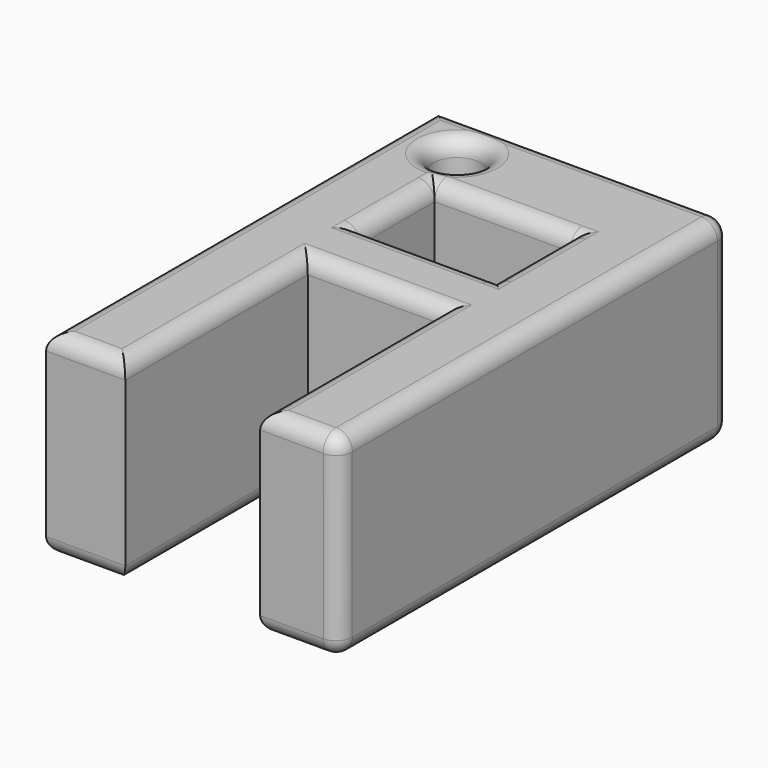
from build123d import *

# Parameters (mm, degrees)
F0_W          = 10.5156756136
F0_H          = 7.2225928307
F1_DEPTH      = 15.24
F2_R          = 1.8806308745
F3_DEPTH      = 25.4
F4_T1_DEPTH   = 24.7648500098
F4_T3_DEPTH   = 35.5602
F4_T5_DEPTH   = 44.4495000197
F4_T7_DEPTH   = 8.0769743963
F4_T9_DEPTH   = 12.5217000197
F4_T11_DEPTH  = 20.9547500098
F4_T13_DEPTH  = 10.5156756136
F4_T15_DEPTH  = 7.2225928307
F4_T17_DEPTH  = 12.7002
F4_S21_W      = 1.2954
F4_S21_H      = 1.2954
F4_T22_DEPTH  = 1.2954
F4_S27_W      = 1.2954
F4_S27_H      = 1.2954
F4_T28_DEPTH  = 1.2954
F4_S33_W      = 1.2954
F4_S33_H      = 1.2954
F4_T34_DEPTH  = 1.2954
F4_S39_W      = 1.2954
F4_S39_H      = 1.2954
F4_T40_DEPTH  = 1.2954
F4_T51_DEPTH  = 24.1295000197
F4_T55_DEPTH  = 13.6904256234
F4_T62_DEPTH  = 24.1295000197
F4_T66_DEPTH  = 13.6904256234
F4_T73_DEPTH  = 13.6904256234
F4_T77_DEPTH  = 10.3973428405
F4_T84_DEPTH  = 13.6904256234
F4_T88_DEPTH  = 10.3973428405
F4_T95_DEPTH  = 10.3973428405
F4_T99_DEPTH  = 13.6904256234
F4_T106_DEPTH = 10.3973428405
F4_T110_DEPTH = 13.6904256234
F4_T117_DEPTH = 24.1295000197
F4_T121_DEPTH = 13.6904256234
F4_T128_DEPTH = 24.1295000197
F4_T132_DEPTH = 13.6904256234
F4_T139_DEPTH = 13.6904256234
F4_T143_DEPTH = 10.3973428405
F4_T150_DEPTH = 13.6904256234
F4_T154_DEPTH = 10.3973428405
F4_T161_DEPTH = 10.3973428405
F4_T165_DEPTH = 13.6904256234
F4_T172_DEPTH = 10.3973428405
F4_T176_DEPTH = 13.6904256234


# Not quite as in the source:
# - a fillet or chamfer that OpenCascade refuses, or shapes differently, is made with other operations: its cross-section is extruded or revolved along the edge and cut away or added


with BuildPart() as f1:
    # F0 (on Top) → F1 (new body)
    with BuildSketch(Plane.XY):
        Polygon((-36.2111851573, 38.1), (-36.2111851573, 0), (-30.0389851573, 0), (-30.0389851573, 17.78), (-19.5233095437, 17.78), (-19.5233095437, 0), (-13.3511851573, 0), (-13.3511851573, 38.1), align=None)
        with Locations((-24.7811473505, 26.5260804445)):
            Rectangle(F0_W, F0_H, mode=Mode.SUBTRACT)
    extrude(amount=F1_DEPTH)

    # F2 (on face) → F3 (cut)
    with BuildSketch(Plane.XY.offset(15.24)):
        with Locations((-31.4282216132, 34.0683087707)):
            Circle(F2_R)
    extrude(amount=-F3_DEPTH, mode=Mode.SUBTRACT)

    # F4: fillet of radius 1.27 on 28 edges, made by hand

    # F4_s2 → F4_t1 (cut)
    with BuildSketch(Plane.YZ.offset(-39.3859351671)):
        with BuildLine():
            ThreePointArc((38.1001, 13.9701), (37.7281256121, 14.8681256121), (36.8301, 15.2401))
            Line((36.8301, 15.2401), (36.8301, 15.2655))
            ThreePointArc((36.8301, 15.2655), (37.46505, 15.2654), (38.1, 15.2654))
            Line((38.1, 15.2654), (38.1254, 15.24))
            ThreePointArc((38.1254, 15.24), (38.1254, 14.60505), (38.1255, 13.9701))
            Line((38.1255, 13.9701), (38.1001, 13.9701))
        make_face()
        with BuildLine():
            ThreePointArc((38.1001, 1.2699), (37.7281256121, 0.3718743879), (36.8301, -0.0001))
            Line((36.8301, -0.0001), (36.8301, -0.0255))
            ThreePointArc((36.8301, -0.0255), (37.46505, -0.0254), (38.1, -0.0254))
            Line((38.1, -0.0254), (38.1254, 0))
            ThreePointArc((38.1254, 0), (38.1254, 0.63495), (38.1255, 1.2699))
            Line((38.1255, 1.2699), (38.1001, 1.2699))
        make_face()
    extrude(amount=F4_T1_DEPTH, mode=Mode.SUBTRACT)

    # F4_s4 → F4_t3 (cut)
    with BuildSketch(Plane.XZ.offset(-36.8301)):
        with BuildLine():
            ThreePointArc((-13.3510851573, 13.9701), (-13.7230595452, 14.8681256121), (-14.6210851573, 15.2401))
            Line((-14.6210851573, 15.2401), (-14.6210851573, 15.2655))
            ThreePointArc((-14.6210851573, 15.2655), (-13.9861351573, 15.2654), (-13.3511851573, 15.2654))
            Line((-13.3511851573, 15.2654), (-13.3257851573, 15.24))
            ThreePointArc((-13.3257851573, 15.24), (-13.3257851573, 14.60505), (-13.3256851573, 13.9701))
            Line((-13.3256851573, 13.9701), (-13.3510851573, 13.9701))
        make_face()
        with BuildLine():
            ThreePointArc((-13.3510851573, 1.2699), (-13.7230595452, 0.3718743879), (-14.6210851573, -0.0001))
            Line((-14.6210851573, -0.0001), (-14.6210851573, -0.0255))
            ThreePointArc((-14.6210851573, -0.0255), (-13.9861351573, -0.0254), (-13.3511851573, -0.0254))
            Line((-13.3511851573, -0.0254), (-13.3257851573, 0))
            ThreePointArc((-13.3257851573, 0), (-13.3257851573, 0.63495), (-13.3256851573, 1.2699))
            Line((-13.3256851573, 1.2699), (-13.3510851573, 1.2699))
        make_face()
    extrude(amount=F4_T3_DEPTH, mode=Mode.SUBTRACT)

    # F4_s6 → F4_t5 (cut)
    with BuildSketch(Plane.XZ.offset(-41.2747500098)):
        with BuildLine():
            ThreePointArc((-36.2112851573, 13.9701), (-35.8393107694, 14.8681256121), (-34.9412851573, 15.2401))
            Line((-34.9412851573, 15.2401), (-34.9412851573, 15.2655))
            ThreePointArc((-34.9412851573, 15.2655), (-35.5762351573, 15.2654), (-36.2111851573, 15.2654))
            Line((-36.2111851573, 15.2654), (-36.2365851573, 15.24))
            ThreePointArc((-36.2365851573, 15.24), (-36.2365851573, 14.60505), (-36.2366851573, 13.9701))
            Line((-36.2366851573, 13.9701), (-36.2112851573, 13.9701))
        make_face()
        with BuildLine():
            ThreePointArc((-36.2112851573, 1.2699), (-35.8393107694, 0.3718743879), (-34.9412851573, -0.0001))
            Line((-34.9412851573, -0.0001), (-34.9412851573, -0.0255))
            ThreePointArc((-34.9412851573, -0.0255), (-35.5762351573, -0.0254), (-36.2111851573, -0.0254))
            Line((-36.2111851573, -0.0254), (-36.2365851573, 0))
            ThreePointArc((-36.2365851573, 0), (-36.2365851573, 0.63495), (-36.2366851573, 1.2699))
            Line((-36.2366851573, 1.2699), (-36.2112851573, 1.2699))
        make_face()
    extrude(amount=F4_T5_DEPTH, mode=Mode.SUBTRACT)

    # F4_s8 → F4_t7 (cut)
    with BuildSketch(Plane.YZ.offset(-22.6980595536)):
        with BuildLine():
            ThreePointArc((1.2699, 15.2401), (0.3718743879, 14.8681256121), (-0.0001, 13.9701))
            Line((-0.0001, 13.9701), (-0.0255, 13.9701))
            ThreePointArc((-0.0255, 13.9701), (-0.0254, 14.60505), (-0.0254, 15.24))
            Line((-0.0254, 15.24), (0, 15.2654))
            ThreePointArc((0, 15.2654), (0.63495, 15.2654), (1.2699, 15.2655))
            Line((1.2699, 15.2655), (1.2699, 15.2401))
        make_face()
        with BuildLine():
            ThreePointArc((1.2699, -0.0001), (0.3718743879, 0.3718743879), (-0.0001, 1.2699))
            Line((-0.0001, 1.2699), (-0.0255, 1.2699))
            ThreePointArc((-0.0255, 1.2699), (-0.0254, 0.63495), (-0.0254, 0))
            Line((-0.0254, 0), (0, -0.0254))
            ThreePointArc((0, -0.0254), (0.63495, -0.0254), (1.2699, -0.0255))
            Line((1.2699, -0.0255), (1.2699, -0.0001))
        make_face()
    extrude(amount=F4_T7_DEPTH, mode=Mode.SUBTRACT)

    # F4_s10 → F4_t9 (cut)
    with BuildSketch(Plane.YZ.offset(-39.3859351671)):
        with BuildLine():
            ThreePointArc((1.2699, 15.2401), (0.3718743879, 14.8681256121), (-0.0001, 13.9701))
            Line((-0.0001, 13.9701), (-0.0255, 13.9701))
            ThreePointArc((-0.0255, 13.9701), (-0.0254, 14.60505), (-0.0254, 15.24))
            Line((-0.0254, 15.24), (0, 15.2654))
            ThreePointArc((0, 15.2654), (0.63495, 15.2654), (1.2699, 15.2655))
            Line((1.2699, 15.2655), (1.2699, 15.2401))
        make_face()
        with BuildLine():
            ThreePointArc((1.2699, -0.0001), (0.3718743879, 0.3718743879), (-0.0001, 1.2699))
            Line((-0.0001, 1.2699), (-0.0255, 1.2699))
            ThreePointArc((-0.0255, 1.2699), (-0.0254, 0.63495), (-0.0254, 0))
            Line((-0.0254, 0), (0, -0.0254))
            ThreePointArc((0, -0.0254), (0.63495, -0.0254), (1.2699, -0.0255))
            Line((1.2699, -0.0255), (1.2699, -0.0001))
        make_face()
    extrude(amount=F4_T9_DEPTH, mode=Mode.SUBTRACT)

    # F4_s12 → F4_t11 (cut)
    with BuildSketch(Plane.XZ.offset(-17.78)):
        with BuildLine():
            ThreePointArc((-18.2534095437, 15.2401), (-19.1514351558, 14.8681256121), (-19.5234095437, 13.9701))
            Line((-19.5234095437, 13.9701), (-19.5488095437, 13.9701))
            ThreePointArc((-19.5488095437, 13.9701), (-19.5487095437, 14.60505), (-19.5487095437, 15.24))
            Line((-19.5487095437, 15.24), (-19.5233095437, 15.2654))
            ThreePointArc((-19.5233095437, 15.2654), (-18.8883595437, 15.2654), (-18.2534095437, 15.2655))
            Line((-18.2534095437, 15.2655), (-18.2534095437, 15.2401))
        make_face()
        with BuildLine():
            ThreePointArc((-31.3088851573, 15.2401), (-30.4108595452, 14.8681256121), (-30.0388851573, 13.9701))
            Line((-30.0388851573, 13.9701), (-30.0134851573, 13.9701))
            ThreePointArc((-30.0134851573, 13.9701), (-30.0135851573, 14.60505), (-30.0135851573, 15.24))
            Line((-30.0135851573, 15.24), (-30.0389851573, 15.2654))
            ThreePointArc((-30.0389851573, 15.2654), (-30.6739351573, 15.2654), (-31.3088851573, 15.2655))
            Line((-31.3088851573, 15.2655), (-31.3088851573, 15.2401))
        make_face()
        with BuildLine():
            ThreePointArc((-18.2534095437, -0.0001), (-19.1514351558, 0.3718743879), (-19.5234095437, 1.2699))
            Line((-19.5234095437, 1.2699), (-19.5488095437, 1.2699))
            ThreePointArc((-19.5488095437, 1.2699), (-19.5487095437, 0.63495), (-19.5487095437, 0))
            Line((-19.5487095437, 0), (-19.5233095437, -0.0254))
            ThreePointArc((-19.5233095437, -0.0254), (-18.8883595437, -0.0254), (-18.2534095437, -0.0255))
            Line((-18.2534095437, -0.0255), (-18.2534095437, -0.0001))
        make_face()
        with BuildLine():
            ThreePointArc((-31.3088851573, -0.0001), (-30.4108595452, 0.3718743879), (-30.0388851573, 1.2699))
            Line((-30.0388851573, 1.2699), (-30.0134851573, 1.2699))
            ThreePointArc((-30.0134851573, 1.2699), (-30.0135851573, 0.63495), (-30.0135851573, 0))
            Line((-30.0135851573, 0), (-30.0389851573, -0.0254))
            ThreePointArc((-30.0389851573, -0.0254), (-30.6739351573, -0.0254), (-31.3088851573, -0.0255))
            Line((-31.3088851573, -0.0255), (-31.3088851573, -0.0001))
        make_face()
    extrude(amount=F4_T11_DEPTH, mode=Mode.SUBTRACT)

    # F4_s14 → F4_t13 (cut)
    with BuildSketch(Plane.YZ.offset(-30.0389851573)):
        with BuildLine():
            ThreePointArc((19.0499, 15.2401), (18.1518743879, 14.8681256121), (17.7799, 13.9701))
            Line((17.7799, 13.9701), (17.7545, 13.9701))
            ThreePointArc((17.7545, 13.9701), (17.7546, 14.60505), (17.7546, 15.24))
            Line((17.7546, 15.24), (17.78, 15.2654))
            ThreePointArc((17.78, 15.2654), (18.41495, 15.2654), (19.0499, 15.2655))
            Line((19.0499, 15.2655), (19.0499, 15.2401))
        make_face()
        with BuildLine():
            ThreePointArc((21.6448840291, 15.2401), (22.5429096412, 14.8681256121), (22.9148840291, 13.9701))
            Line((22.9148840291, 13.9701), (22.9402840291, 13.9701))
            ThreePointArc((22.9402840291, 13.9701), (22.9401840291, 14.60505), (22.9401840291, 15.24))
            Line((22.9401840291, 15.24), (22.9147840291, 15.2654))
            ThreePointArc((22.9147840291, 15.2654), (22.2798340291, 15.2654), (21.6448840291, 15.2655))
            Line((21.6448840291, 15.2655), (21.6448840291, 15.2401))
        make_face()
        with BuildLine():
            ThreePointArc((31.4072768598, 15.2401), (30.5092512477, 14.8681256121), (30.1372768598, 13.9701))
            Line((30.1372768598, 13.9701), (30.1118768598, 13.9701))
            ThreePointArc((30.1118768598, 13.9701), (30.1119768598, 14.60505), (30.1119768598, 15.24))
            Line((30.1119768598, 15.24), (30.1373768598, 15.2654))
            ThreePointArc((30.1373768598, 15.2654), (30.7723268598, 15.2654), (31.4072768598, 15.2655))
            Line((31.4072768598, 15.2655), (31.4072768598, 15.2401))
        make_face()
        with BuildLine():
            ThreePointArc((19.0499, -0.0001), (18.1518743879, 0.3718743879), (17.7799, 1.2699))
            Line((17.7799, 1.2699), (17.7545, 1.2699))
            ThreePointArc((17.7545, 1.2699), (17.7546, 0.63495), (17.7546, 0))
            Line((17.7546, 0), (17.78, -0.0254))
            ThreePointArc((17.78, -0.0254), (18.41495, -0.0254), (19.0499, -0.0255))
            Line((19.0499, -0.0255), (19.0499, -0.0001))
        make_face()
        with BuildLine():
            ThreePointArc((21.6448840291, -0.0001), (22.5429096412, 0.3718743879), (22.9148840291, 1.2699))
            Line((22.9148840291, 1.2699), (22.9402840291, 1.2699))
            ThreePointArc((22.9402840291, 1.2699), (22.9401840291, 0.63495), (22.9401840291, 0))
            Line((22.9401840291, 0), (22.9147840291, -0.0254))
            ThreePointArc((22.9147840291, -0.0254), (22.2798340291, -0.0254), (21.6448840291, -0.0255))
            Line((21.6448840291, -0.0255), (21.6448840291, -0.0001))
        make_face()
        with BuildLine():
            ThreePointArc((31.4072768598, -0.0001), (30.5092512477, 0.3718743879), (30.1372768598, 1.2699))
            Line((30.1372768598, 1.2699), (30.1118768598, 1.2699))
            ThreePointArc((30.1118768598, 1.2699), (30.1119768598, 0.63495), (30.1119768598, 0))
            Line((30.1119768598, 0), (30.1373768598, -0.0254))
            ThreePointArc((30.1373768598, -0.0254), (30.7723268598, -0.0254), (31.4072768598, -0.0255))
            Line((31.4072768598, -0.0255), (31.4072768598, -0.0001))
        make_face()
    extrude(amount=F4_T13_DEPTH, mode=Mode.SUBTRACT)

    # F4_s16 → F4_t15 (cut)
    with BuildSketch(Plane.XZ.offset(-30.1373768598)):
        with BuildLine():
            ThreePointArc((-18.2534095437, 15.2401), (-19.1514351558, 14.8681256121), (-19.5234095437, 13.9701))
            Line((-19.5234095437, 13.9701), (-19.5488095437, 13.9701))
            ThreePointArc((-19.5488095437, 13.9701), (-19.5487095437, 14.60505), (-19.5487095437, 15.24))
            Line((-19.5487095437, 15.24), (-19.5233095437, 15.2654))
            ThreePointArc((-19.5233095437, 15.2654), (-18.8883595437, 15.2654), (-18.2534095437, 15.2655))
            Line((-18.2534095437, 15.2655), (-18.2534095437, 15.2401))
        make_face()
        with BuildLine():
            ThreePointArc((-31.3088851573, 15.2401), (-30.4108595452, 14.8681256121), (-30.0388851573, 13.9701))
            Line((-30.0388851573, 13.9701), (-30.0134851573, 13.9701))
            ThreePointArc((-30.0134851573, 13.9701), (-30.0135851573, 14.60505), (-30.0135851573, 15.24))
            Line((-30.0135851573, 15.24), (-30.0389851573, 15.2654))
            ThreePointArc((-30.0389851573, 15.2654), (-30.6739351573, 15.2654), (-31.3088851573, 15.2655))
            Line((-31.3088851573, 15.2655), (-31.3088851573, 15.2401))
        make_face()
        with BuildLine():
            ThreePointArc((-18.2534095437, -0.0001), (-19.1514351558, 0.3718743879), (-19.5234095437, 1.2699))
            Line((-19.5234095437, 1.2699), (-19.5488095437, 1.2699))
            ThreePointArc((-19.5488095437, 1.2699), (-19.5487095437, 0.63495), (-19.5487095437, 0))
            Line((-19.5487095437, 0), (-19.5233095437, -0.0254))
            ThreePointArc((-19.5233095437, -0.0254), (-18.8883595437, -0.0254), (-18.2534095437, -0.0255))
            Line((-18.2534095437, -0.0255), (-18.2534095437, -0.0001))
        make_face()
        with BuildLine():
            ThreePointArc((-31.3088851573, -0.0001), (-30.4108595452, 0.3718743879), (-30.0388851573, 1.2699))
            Line((-30.0388851573, 1.2699), (-30.0134851573, 1.2699))
            ThreePointArc((-30.0134851573, 1.2699), (-30.0135851573, 0.63495), (-30.0135851573, 0))
            Line((-30.0135851573, 0), (-30.0389851573, -0.0254))
            ThreePointArc((-30.0389851573, -0.0254), (-30.6739351573, -0.0254), (-31.3088851573, -0.0255))
            Line((-31.3088851573, -0.0255), (-31.3088851573, -0.0001))
        make_face()
    extrude(amount=F4_T15_DEPTH, mode=Mode.SUBTRACT)

    # F4_s18 → F4_t17 (cut)
    with BuildSketch(Plane.XY.offset(1.2699)):
        with BuildLine():
            ThreePointArc((-13.3510851573, 1.2699), (-13.7230595452, 0.3718743879), (-14.6210851573, -0.0001))
            Line((-14.6210851573, -0.0001), (-14.6210851573, -0.0255))
            ThreePointArc((-14.6210851573, -0.0255), (-13.9861351573, -0.0254), (-13.3511851573, -0.0254))
            Line((-13.3511851573, -0.0254), (-13.3257851573, 0))
            ThreePointArc((-13.3257851573, 0), (-13.3257851573, 0.63495), (-13.3256851573, 1.2699))
            Line((-13.3256851573, 1.2699), (-13.3510851573, 1.2699))
        make_face()
        with BuildLine():
            ThreePointArc((-14.6210851573, 38.1001), (-13.7230595452, 37.7281256121), (-13.3510851573, 36.8301))
            Line((-13.3510851573, 36.8301), (-13.3256851573, 36.8301))
            ThreePointArc((-13.3256851573, 36.8301), (-13.3257851573, 37.46505), (-13.3257851573, 38.1))
            Line((-13.3257851573, 38.1), (-13.3511851573, 38.1254))
            ThreePointArc((-13.3511851573, 38.1254), (-13.9861351573, 38.1254), (-14.6210851573, 38.1255))
            Line((-14.6210851573, 38.1255), (-14.6210851573, 38.1001))
        make_face()
    extrude(amount=F4_T17_DEPTH, mode=Mode.SUBTRACT)


with BuildPart() as f4_tool20:
    # F4_s21 → F4_t22 (new body)
    with BuildSketch(Plane.XZ.offset(-36.8301)):
        with Locations((-13.9733851573, 14.6178)):
            Rectangle(F4_S21_W, F4_S21_H)
    extrude(amount=-F4_T22_DEPTH)

    # F4_s23 → F4_t24 (revolve, cut)
    with BuildSketch(Plane(origin=(-14.6210851573, 36.8301, 13.9701), x_dir=(-0.7071067812, 0, -0.7071067812), z_dir=(0.7071067812, 0, -0.7071067812))):
        with BuildLine():
            ThreePointArc((0, -1.27), (1.27, 0), (0, 1.27))
            Line((0, 1.27), (0, -1.27))
        make_face()
    revolve(axis=Axis((-14.6210851573, 36.8301, 13.9701), (0, 1, 0)), mode=Mode.SUBTRACT)


with BuildPart() as f1_1:
    add(f1.part)

    # F4_t19: cut F4_tool20
    add(f4_tool20.part, mode=Mode.SUBTRACT)


with BuildPart() as f4_tool26:
    # F4_s27 → F4_t28 (new body)
    with BuildSketch(Plane.YZ.offset(-14.6210851573)):
        with Locations((0.6222, 14.6178)):
            Rectangle(F4_S27_W, F4_S27_H)
    extrude(amount=F4_T28_DEPTH)

    # F4_s29 → F4_t30 (revolve, cut)
    with BuildSketch(Plane(origin=(-14.6210851573, 1.2699, 13.9701), x_dir=(0, 0.7071067812, -0.7071067812), z_dir=(0, -0.7071067812, -0.7071067812))):
        with BuildLine():
            ThreePointArc((0, -1.27), (1.27, 0), (0, 1.27))
            Line((0, 1.27), (0, -1.27))
        make_face()
    revolve(axis=Axis((-14.6210851573, 1.2699, 13.9701), (1, 0, 0)), mode=Mode.SUBTRACT)


with BuildPart() as f1_2:
    add(f1_1.part)

    # F4_t25: cut F4_tool26
    add(f4_tool26.part, mode=Mode.SUBTRACT)


with BuildPart() as f4_tool32:
    # F4_s33 → F4_t34 (new body)
    with BuildSketch(Plane.XZ.offset(-36.8301)):
        with Locations((-13.9733851573, 0.6222)):
            Rectangle(F4_S33_W, F4_S33_H)
    extrude(amount=-F4_T34_DEPTH)

    # F4_s35 → F4_t36 (revolve, cut)
    with BuildSketch(Plane(origin=(-14.6210851573, 36.8301, 1.2699), x_dir=(-0.7071067812, 0, 0.7071067812), z_dir=(-0.7071067812, 0, -0.7071067812))):
        with BuildLine():
            ThreePointArc((0, -1.27), (1.27, 0), (0, 1.27))
            Line((0, 1.27), (0, -1.27))
        make_face()
    revolve(axis=Axis((-14.6210851573, 36.8301, 1.2699), (0, 1, 0)), mode=Mode.SUBTRACT)


with BuildPart() as f1_3:
    add(f1_2.part)

    # F4_t31: cut F4_tool32
    add(f4_tool32.part, mode=Mode.SUBTRACT)


with BuildPart() as f4_tool38:
    # F4_s39 → F4_t40 (new body)
    with BuildSketch(Plane.YZ.offset(-14.6210851573)):
        with Locations((0.6222, 0.6222)):
            Rectangle(F4_S39_W, F4_S39_H)
    extrude(amount=F4_T40_DEPTH)

    # F4_s41 → F4_t42 (revolve, cut)
    with BuildSketch(Plane(origin=(-14.6210851573, 1.2699, 1.2699), x_dir=(0, 0.7071067812, 0.7071067812), z_dir=(0, 0.7071067812, -0.7071067812))):
        with BuildLine():
            ThreePointArc((0, -1.27), (1.27, 0), (0, 1.27))
            Line((0, 1.27), (0, -1.27))
        make_face()
    revolve(axis=Axis((-14.6210851573, 1.2699, 1.2699), (1, 0, 0)), mode=Mode.SUBTRACT)


with BuildPart() as f1_4:
    add(f1_3.part)

    # F4_t37: cut F4_tool38
    add(f4_tool38.part, mode=Mode.SUBTRACT)

    # F4_s43 → F4_t44 (revolve, cut)
    with BuildSketch(Plane.XZ.offset(-34.0683087707)):
        with BuildLine():
            ThreePointArc((-28.2776907386, 15.2401), (-29.1757163507, 14.8681256121), (-29.5476907386, 13.9701))
            Line((-29.5476907386, 13.9701), (-29.5730907386, 13.9701))
            ThreePointArc((-29.5730907386, 13.9701), (-29.5729907386, 14.60505), (-29.5729907386, 15.24))
            Line((-29.5729907386, 15.24), (-29.5475907386, 15.2654))
            ThreePointArc((-29.5475907386, 15.2654), (-28.9126407386, 15.2654), (-28.2776907386, 15.2655))
            Line((-28.2776907386, 15.2655), (-28.2776907386, 15.2401))
        make_face()
    revolve(axis=Axis((-31.4282216132, 34.0683087707, 15.24), (0, 0, 1)), mode=Mode.SUBTRACT)

    # F4_s45 → F4_t46 (revolve, cut)
    with BuildSketch(Plane.XZ.offset(-34.0683087707)):
        with BuildLine():
            ThreePointArc((-28.2776907386, -0.0001), (-29.1757163507, 0.3718743879), (-29.5476907386, 1.2699))
            Line((-29.5476907386, 1.2699), (-29.5730907386, 1.2699))
            ThreePointArc((-29.5730907386, 1.2699), (-29.5729907386, 0.63495), (-29.5729907386, 0))
            Line((-29.5729907386, 0), (-29.5475907386, -0.0254))
            ThreePointArc((-29.5475907386, -0.0254), (-28.9126407386, -0.0254), (-28.2776907386, -0.0255))
            Line((-28.2776907386, -0.0255), (-28.2776907386, -0.0001))
        make_face()
    revolve(axis=Axis((-31.4282216132, 34.0683087707, 0), (0, 0, 1)), mode=Mode.SUBTRACT)


with BuildPart() as f4_tool49:
    # F4_s50 → F4_t51 (new body)
    with BuildSketch(Plane.XZ.offset(-20.9547500098)):
        with BuildLine():
            ThreePointArc((-18.2534095437, 15.2401), (-19.1514351558, 14.8681256121), (-19.5234095437, 13.9701))
            Line((-19.5234095437, 13.9701), (-19.5488095437, 13.9701))
            ThreePointArc((-19.5488095437, 13.9701), (-19.5487095437, 14.60505), (-19.5487095437, 15.24))
            Line((-19.5487095437, 15.24), (-19.5233095437, 15.2654))
            ThreePointArc((-19.5233095437, 15.2654), (-18.8883595437, 15.2654), (-18.2534095437, 15.2655))
            Line((-18.2534095437, 15.2655), (-18.2534095437, 15.2401))
        make_face()
    extrude(amount=F4_T51_DEPTH)

    split(bisect_by=Plane.XZ.offset(-17.78), keep=Keep.BOTTOM)


with BuildPart() as f4_tool53:
    # F4_s54 → F4_t55 (new body)
    with BuildSketch(Plane.YZ.offset(-30.0389851573)):
        with BuildLine():
            ThreePointArc((19.0499, 15.2401), (18.1518743879, 14.8681256121), (17.7799, 13.9701))
            Line((17.7799, 13.9701), (17.7545, 13.9701))
            ThreePointArc((17.7545, 13.9701), (17.7546, 14.60505), (17.7546, 15.24))
            Line((17.7546, 15.24), (17.78, 15.2654))
            ThreePointArc((17.78, 15.2654), (18.41495, 15.2654), (19.0499, 15.2655))
            Line((19.0499, 15.2655), (19.0499, 15.2401))
        make_face()
    extrude(amount=F4_T55_DEPTH)

    split(bisect_by=Plane.YZ.offset(-19.5233095437), keep=Keep.TOP)


with BuildPart() as f4_tool49_1:
    add(f4_tool49.part)

    # F4_t57: intersect F4_tool53
    add(f4_tool53.part, mode=Mode.INTERSECT)


with BuildPart() as f1_5:
    add(f1_4.part)

    # F4_t47: cut F4_tool49
    add(f4_tool49_1.part, mode=Mode.SUBTRACT)


with BuildPart() as f4_tool60:
    # F4_s61 → F4_t62 (new body)
    with BuildSketch(Plane.XZ.offset(3.1747500098)):
        with BuildLine():
            ThreePointArc((-31.3088851573, 15.2401), (-30.4108595452, 14.8681256121), (-30.0388851573, 13.9701))
            Line((-30.0388851573, 13.9701), (-30.0134851573, 13.9701))
            ThreePointArc((-30.0134851573, 13.9701), (-30.0135851573, 14.60505), (-30.0135851573, 15.24))
            Line((-30.0135851573, 15.24), (-30.0389851573, 15.2654))
            ThreePointArc((-30.0389851573, 15.2654), (-30.6739351573, 15.2654), (-31.3088851573, 15.2655))
            Line((-31.3088851573, 15.2655), (-31.3088851573, 15.2401))
        make_face()
    extrude(amount=-F4_T62_DEPTH)

    split(bisect_by=Plane.XZ.offset(-17.78), keep=Keep.BOTTOM)


with BuildPart() as f4_tool64:
    # F4_s65 → F4_t66 (new body)
    with BuildSketch(Plane.YZ.offset(-33.2137351671)):
        with BuildLine():
            ThreePointArc((19.0499, 15.2401), (18.1518743879, 14.8681256121), (17.7799, 13.9701))
            Line((17.7799, 13.9701), (17.7545, 13.9701))
            ThreePointArc((17.7545, 13.9701), (17.7546, 14.60505), (17.7546, 15.24))
            Line((17.7546, 15.24), (17.78, 15.2654))
            ThreePointArc((17.78, 15.2654), (18.41495, 15.2654), (19.0499, 15.2655))
            Line((19.0499, 15.2655), (19.0499, 15.2401))
        make_face()
    extrude(amount=F4_T66_DEPTH)

    split(bisect_by=Plane.YZ.offset(-30.0389851573), keep=Keep.BOTTOM)


with BuildPart() as f4_tool60_1:
    add(f4_tool60.part)

    # F4_t68: intersect F4_tool64
    add(f4_tool64.part, mode=Mode.INTERSECT)


with BuildPart() as f1_6:
    add(f1_5.part)

    # F4_t58: cut F4_tool60
    add(f4_tool60_1.part, mode=Mode.SUBTRACT)


with BuildPart() as f4_tool71:
    # F4_s72 → F4_t73 (new body)
    with BuildSketch(Plane.YZ.offset(-16.3485595339)):
        with BuildLine():
            ThreePointArc((21.6448840291, 15.2401), (22.5429096412, 14.8681256121), (22.9148840291, 13.9701))
            Line((22.9148840291, 13.9701), (22.9402840291, 13.9701))
            ThreePointArc((22.9402840291, 13.9701), (22.9401840291, 14.60505), (22.9401840291, 15.24))
            Line((22.9401840291, 15.24), (22.9147840291, 15.2654))
            ThreePointArc((22.9147840291, 15.2654), (22.2798340291, 15.2654), (21.6448840291, 15.2655))
            Line((21.6448840291, 15.2655), (21.6448840291, 15.2401))
        make_face()
    extrude(amount=-F4_T73_DEPTH)

    split(bisect_by=Plane.YZ.offset(-19.5233095437), keep=Keep.TOP)


with BuildPart() as f4_tool75:
    # F4_s76 → F4_t77 (new body)
    with BuildSketch(Plane.XZ.offset(-30.1373768598)):
        with BuildLine():
            ThreePointArc((-18.2534095437, 15.2401), (-19.1514351558, 14.8681256121), (-19.5234095437, 13.9701))
            Line((-19.5234095437, 13.9701), (-19.5488095437, 13.9701))
            ThreePointArc((-19.5488095437, 13.9701), (-19.5487095437, 14.60505), (-19.5487095437, 15.24))
            Line((-19.5487095437, 15.24), (-19.5233095437, 15.2654))
            ThreePointArc((-19.5233095437, 15.2654), (-18.8883595437, 15.2654), (-18.2534095437, 15.2655))
            Line((-18.2534095437, 15.2655), (-18.2534095437, 15.2401))
        make_face()
    extrude(amount=F4_T77_DEPTH)

    split(bisect_by=Plane.XZ.offset(-22.9147840291), keep=Keep.TOP)


with BuildPart() as f4_tool71_1:
    add(f4_tool71.part)

    # F4_t79: intersect F4_tool75
    add(f4_tool75.part, mode=Mode.INTERSECT)


with BuildPart() as f1_7:
    add(f1_6.part)

    # F4_t69: cut F4_tool71
    add(f4_tool71_1.part, mode=Mode.SUBTRACT)


with BuildPart() as f4_tool82:
    # F4_s83 → F4_t84 (new body)
    with BuildSketch(Plane.YZ.offset(-19.5233095437)):
        with BuildLine():
            ThreePointArc((21.6448840291, 15.2401), (22.5429096412, 14.8681256121), (22.9148840291, 13.9701))
            Line((22.9148840291, 13.9701), (22.9402840291, 13.9701))
            ThreePointArc((22.9402840291, 13.9701), (22.9401840291, 14.60505), (22.9401840291, 15.24))
            Line((22.9401840291, 15.24), (22.9147840291, 15.2654))
            ThreePointArc((22.9147840291, 15.2654), (22.2798340291, 15.2654), (21.6448840291, 15.2655))
            Line((21.6448840291, 15.2655), (21.6448840291, 15.2401))
        make_face()
    extrude(amount=-F4_T84_DEPTH)

    split(bisect_by=Plane.YZ.offset(-30.0389851573), keep=Keep.BOTTOM)


with BuildPart() as f4_tool86:
    # F4_s87 → F4_t88 (new body)
    with BuildSketch(Plane.XZ.offset(-19.7400340193)):
        with BuildLine():
            ThreePointArc((-31.3088851573, 15.2401), (-30.4108595452, 14.8681256121), (-30.0388851573, 13.9701))
            Line((-30.0388851573, 13.9701), (-30.0134851573, 13.9701))
            ThreePointArc((-30.0134851573, 13.9701), (-30.0135851573, 14.60505), (-30.0135851573, 15.24))
            Line((-30.0135851573, 15.24), (-30.0389851573, 15.2654))
            ThreePointArc((-30.0389851573, 15.2654), (-30.6739351573, 15.2654), (-31.3088851573, 15.2655))
            Line((-31.3088851573, 15.2655), (-31.3088851573, 15.2401))
        make_face()
    extrude(amount=-F4_T88_DEPTH)

    split(bisect_by=Plane.XZ.offset(-22.9147840291), keep=Keep.TOP)


with BuildPart() as f4_tool82_1:
    add(f4_tool82.part)

    # F4_t90: intersect F4_tool86
    add(f4_tool86.part, mode=Mode.INTERSECT)


with BuildPart() as f1_8:
    add(f1_7.part)

    # F4_t80: cut F4_tool82
    add(f4_tool82_1.part, mode=Mode.SUBTRACT)


with BuildPart() as f4_tool93:
    # F4_s94 → F4_t95 (new body)
    with BuildSketch(Plane.XZ.offset(-33.3121268696)):
        with BuildLine():
            ThreePointArc((-18.2534095437, 15.2401), (-19.1514351558, 14.8681256121), (-19.5234095437, 13.9701))
            Line((-19.5234095437, 13.9701), (-19.5488095437, 13.9701))
            ThreePointArc((-19.5488095437, 13.9701), (-19.5487095437, 14.60505), (-19.5487095437, 15.24))
            Line((-19.5487095437, 15.24), (-19.5233095437, 15.2654))
            ThreePointArc((-19.5233095437, 15.2654), (-18.8883595437, 15.2654), (-18.2534095437, 15.2655))
            Line((-18.2534095437, 15.2655), (-18.2534095437, 15.2401))
        make_face()
    extrude(amount=F4_T95_DEPTH)

    split(bisect_by=Plane.XZ.offset(-30.1373768598), keep=Keep.BOTTOM)


with BuildPart() as f4_tool97:
    # F4_s98 → F4_t99 (new body)
    with BuildSketch(Plane.YZ.offset(-30.0389851573)):
        with BuildLine():
            ThreePointArc((31.4072768598, 15.2401), (30.5092512477, 14.8681256121), (30.1372768598, 13.9701))
            Line((30.1372768598, 13.9701), (30.1118768598, 13.9701))
            ThreePointArc((30.1118768598, 13.9701), (30.1119768598, 14.60505), (30.1119768598, 15.24))
            Line((30.1119768598, 15.24), (30.1373768598, 15.2654))
            ThreePointArc((30.1373768598, 15.2654), (30.7723268598, 15.2654), (31.4072768598, 15.2655))
            Line((31.4072768598, 15.2655), (31.4072768598, 15.2401))
        make_face()
    extrude(amount=F4_T99_DEPTH)

    split(bisect_by=Plane.YZ.offset(-19.5233095437), keep=Keep.TOP)


with BuildPart() as f4_tool93_1:
    add(f4_tool93.part)

    # F4_t101: intersect F4_tool97
    add(f4_tool97.part, mode=Mode.INTERSECT)


with BuildPart() as f1_9:
    add(f1_8.part)

    # F4_t91: cut F4_tool93
    add(f4_tool93_1.part, mode=Mode.SUBTRACT)


with BuildPart() as f4_tool104:
    # F4_s105 → F4_t106 (new body)
    with BuildSketch(Plane.XZ.offset(-22.9147840291)):
        with BuildLine():
            ThreePointArc((-31.3088851573, 15.2401), (-30.4108595452, 14.8681256121), (-30.0388851573, 13.9701))
            Line((-30.0388851573, 13.9701), (-30.0134851573, 13.9701))
            ThreePointArc((-30.0134851573, 13.9701), (-30.0135851573, 14.60505), (-30.0135851573, 15.24))
            Line((-30.0135851573, 15.24), (-30.0389851573, 15.2654))
            ThreePointArc((-30.0389851573, 15.2654), (-30.6739351573, 15.2654), (-31.3088851573, 15.2655))
            Line((-31.3088851573, 15.2655), (-31.3088851573, 15.2401))
        make_face()
    extrude(amount=-F4_T106_DEPTH)

    split(bisect_by=Plane.XZ.offset(-30.1373768598), keep=Keep.BOTTOM)


with BuildPart() as f4_tool108:
    # F4_s109 → F4_t110 (new body)
    with BuildSketch(Plane.YZ.offset(-33.2137351671)):
        with BuildLine():
            ThreePointArc((31.4072768598, 15.2401), (30.5092512477, 14.8681256121), (30.1372768598, 13.9701))
            Line((30.1372768598, 13.9701), (30.1118768598, 13.9701))
            ThreePointArc((30.1118768598, 13.9701), (30.1119768598, 14.60505), (30.1119768598, 15.24))
            Line((30.1119768598, 15.24), (30.1373768598, 15.2654))
            ThreePointArc((30.1373768598, 15.2654), (30.7723268598, 15.2654), (31.4072768598, 15.2655))
            Line((31.4072768598, 15.2655), (31.4072768598, 15.2401))
        make_face()
    extrude(amount=F4_T110_DEPTH)

    split(bisect_by=Plane.YZ.offset(-30.0389851573), keep=Keep.BOTTOM)


with BuildPart() as f4_tool104_1:
    add(f4_tool104.part)

    # F4_t112: intersect F4_tool108
    add(f4_tool108.part, mode=Mode.INTERSECT)


with BuildPart() as f1_10:
    add(f1_9.part)

    # F4_t102: cut F4_tool104
    add(f4_tool104_1.part, mode=Mode.SUBTRACT)


with BuildPart() as f4_tool115:
    # F4_s116 → F4_t117 (new body)
    with BuildSketch(Plane.XZ.offset(-20.9547500098)):
        with BuildLine():
            ThreePointArc((-18.2534095437, -0.0001), (-19.1514351558, 0.3718743879), (-19.5234095437, 1.2699))
            Line((-19.5234095437, 1.2699), (-19.5488095437, 1.2699))
            ThreePointArc((-19.5488095437, 1.2699), (-19.5487095437, 0.63495), (-19.5487095437, 0))
            Line((-19.5487095437, 0), (-19.5233095437, -0.0254))
            ThreePointArc((-19.5233095437, -0.0254), (-18.8883595437, -0.0254), (-18.2534095437, -0.0255))
            Line((-18.2534095437, -0.0255), (-18.2534095437, -0.0001))
        make_face()
    extrude(amount=F4_T117_DEPTH)

    split(bisect_by=Plane.XZ.offset(-17.78), keep=Keep.BOTTOM)


with BuildPart() as f4_tool119:
    # F4_s120 → F4_t121 (new body)
    with BuildSketch(Plane.YZ.offset(-30.0389851573)):
        with BuildLine():
            ThreePointArc((19.0499, -0.0001), (18.1518743879, 0.3718743879), (17.7799, 1.2699))
            Line((17.7799, 1.2699), (17.7545, 1.2699))
            ThreePointArc((17.7545, 1.2699), (17.7546, 0.63495), (17.7546, 0))
            Line((17.7546, 0), (17.78, -0.0254))
            ThreePointArc((17.78, -0.0254), (18.41495, -0.0254), (19.0499, -0.0255))
            Line((19.0499, -0.0255), (19.0499, -0.0001))
        make_face()
    extrude(amount=F4_T121_DEPTH)

    split(bisect_by=Plane.YZ.offset(-19.5233095437), keep=Keep.TOP)


with BuildPart() as f4_tool115_1:
    add(f4_tool115.part)

    # F4_t123: intersect F4_tool119
    add(f4_tool119.part, mode=Mode.INTERSECT)


with BuildPart() as f1_11:
    add(f1_10.part)

    # F4_t113: cut F4_tool115
    add(f4_tool115_1.part, mode=Mode.SUBTRACT)


with BuildPart() as f4_tool126:
    # F4_s127 → F4_t128 (new body)
    with BuildSketch(Plane.XZ.offset(3.1747500098)):
        with BuildLine():
            ThreePointArc((-31.3088851573, -0.0001), (-30.4108595452, 0.3718743879), (-30.0388851573, 1.2699))
            Line((-30.0388851573, 1.2699), (-30.0134851573, 1.2699))
            ThreePointArc((-30.0134851573, 1.2699), (-30.0135851573, 0.63495), (-30.0135851573, 0))
            Line((-30.0135851573, 0), (-30.0389851573, -0.0254))
            ThreePointArc((-30.0389851573, -0.0254), (-30.6739351573, -0.0254), (-31.3088851573, -0.0255))
            Line((-31.3088851573, -0.0255), (-31.3088851573, -0.0001))
        make_face()
    extrude(amount=-F4_T128_DEPTH)

    split(bisect_by=Plane.XZ.offset(-17.78), keep=Keep.BOTTOM)


with BuildPart() as f4_tool130:
    # F4_s131 → F4_t132 (new body)
    with BuildSketch(Plane.YZ.offset(-33.2137351671)):
        with BuildLine():
            ThreePointArc((19.0499, -0.0001), (18.1518743879, 0.3718743879), (17.7799, 1.2699))
            Line((17.7799, 1.2699), (17.7545, 1.2699))
            ThreePointArc((17.7545, 1.2699), (17.7546, 0.63495), (17.7546, 0))
            Line((17.7546, 0), (17.78, -0.0254))
            ThreePointArc((17.78, -0.0254), (18.41495, -0.0254), (19.0499, -0.0255))
            Line((19.0499, -0.0255), (19.0499, -0.0001))
        make_face()
    extrude(amount=F4_T132_DEPTH)

    split(bisect_by=Plane.YZ.offset(-30.0389851573), keep=Keep.BOTTOM)


with BuildPart() as f4_tool126_1:
    add(f4_tool126.part)

    # F4_t134: intersect F4_tool130
    add(f4_tool130.part, mode=Mode.INTERSECT)


with BuildPart() as f1_12:
    add(f1_11.part)

    # F4_t124: cut F4_tool126
    add(f4_tool126_1.part, mode=Mode.SUBTRACT)


with BuildPart() as f4_tool137:
    # F4_s138 → F4_t139 (new body)
    with BuildSketch(Plane.YZ.offset(-16.3485595339)):
        with BuildLine():
            ThreePointArc((21.6448840291, -0.0001), (22.5429096412, 0.3718743879), (22.9148840291, 1.2699))
            Line((22.9148840291, 1.2699), (22.9402840291, 1.2699))
            ThreePointArc((22.9402840291, 1.2699), (22.9401840291, 0.63495), (22.9401840291, 0))
            Line((22.9401840291, 0), (22.9147840291, -0.0254))
            ThreePointArc((22.9147840291, -0.0254), (22.2798340291, -0.0254), (21.6448840291, -0.0255))
            Line((21.6448840291, -0.0255), (21.6448840291, -0.0001))
        make_face()
    extrude(amount=-F4_T139_DEPTH)

    split(bisect_by=Plane.YZ.offset(-19.5233095437), keep=Keep.TOP)


with BuildPart() as f4_tool141:
    # F4_s142 → F4_t143 (new body)
    with BuildSketch(Plane.XZ.offset(-30.1373768598)):
        with BuildLine():
            ThreePointArc((-18.2534095437, -0.0001), (-19.1514351558, 0.3718743879), (-19.5234095437, 1.2699))
            Line((-19.5234095437, 1.2699), (-19.5488095437, 1.2699))
            ThreePointArc((-19.5488095437, 1.2699), (-19.5487095437, 0.63495), (-19.5487095437, 0))
            Line((-19.5487095437, 0), (-19.5233095437, -0.0254))
            ThreePointArc((-19.5233095437, -0.0254), (-18.8883595437, -0.0254), (-18.2534095437, -0.0255))
            Line((-18.2534095437, -0.0255), (-18.2534095437, -0.0001))
        make_face()
    extrude(amount=F4_T143_DEPTH)

    split(bisect_by=Plane.XZ.offset(-22.9147840291), keep=Keep.TOP)


with BuildPart() as f4_tool137_1:
    add(f4_tool137.part)

    # F4_t145: intersect F4_tool141
    add(f4_tool141.part, mode=Mode.INTERSECT)


with BuildPart() as f1_13:
    add(f1_12.part)

    # F4_t135: cut F4_tool137
    add(f4_tool137_1.part, mode=Mode.SUBTRACT)


with BuildPart() as f4_tool148:
    # F4_s149 → F4_t150 (new body)
    with BuildSketch(Plane.YZ.offset(-19.5233095437)):
        with BuildLine():
            ThreePointArc((21.6448840291, -0.0001), (22.5429096412, 0.3718743879), (22.9148840291, 1.2699))
            Line((22.9148840291, 1.2699), (22.9402840291, 1.2699))
            ThreePointArc((22.9402840291, 1.2699), (22.9401840291, 0.63495), (22.9401840291, 0))
            Line((22.9401840291, 0), (22.9147840291, -0.0254))
            ThreePointArc((22.9147840291, -0.0254), (22.2798340291, -0.0254), (21.6448840291, -0.0255))
            Line((21.6448840291, -0.0255), (21.6448840291, -0.0001))
        make_face()
    extrude(amount=-F4_T150_DEPTH)

    split(bisect_by=Plane.YZ.offset(-30.0389851573), keep=Keep.BOTTOM)


with BuildPart() as f4_tool152:
    # F4_s153 → F4_t154 (new body)
    with BuildSketch(Plane.XZ.offset(-19.7400340193)):
        with BuildLine():
            ThreePointArc((-31.3088851573, -0.0001), (-30.4108595452, 0.3718743879), (-30.0388851573, 1.2699))
            Line((-30.0388851573, 1.2699), (-30.0134851573, 1.2699))
            ThreePointArc((-30.0134851573, 1.2699), (-30.0135851573, 0.63495), (-30.0135851573, 0))
            Line((-30.0135851573, 0), (-30.0389851573, -0.0254))
            ThreePointArc((-30.0389851573, -0.0254), (-30.6739351573, -0.0254), (-31.3088851573, -0.0255))
            Line((-31.3088851573, -0.0255), (-31.3088851573, -0.0001))
        make_face()
    extrude(amount=-F4_T154_DEPTH)

    split(bisect_by=Plane.XZ.offset(-22.9147840291), keep=Keep.TOP)


with BuildPart() as f4_tool148_1:
    add(f4_tool148.part)

    # F4_t156: intersect F4_tool152
    add(f4_tool152.part, mode=Mode.INTERSECT)


with BuildPart() as f1_14:
    add(f1_13.part)

    # F4_t146: cut F4_tool148
    add(f4_tool148_1.part, mode=Mode.SUBTRACT)


with BuildPart() as f4_tool159:
    # F4_s160 → F4_t161 (new body)
    with BuildSketch(Plane.XZ.offset(-33.3121268696)):
        with BuildLine():
            ThreePointArc((-18.2534095437, -0.0001), (-19.1514351558, 0.3718743879), (-19.5234095437, 1.2699))
            Line((-19.5234095437, 1.2699), (-19.5488095437, 1.2699))
            ThreePointArc((-19.5488095437, 1.2699), (-19.5487095437, 0.63495), (-19.5487095437, 0))
            Line((-19.5487095437, 0), (-19.5233095437, -0.0254))
            ThreePointArc((-19.5233095437, -0.0254), (-18.8883595437, -0.0254), (-18.2534095437, -0.0255))
            Line((-18.2534095437, -0.0255), (-18.2534095437, -0.0001))
        make_face()
    extrude(amount=F4_T161_DEPTH)

    split(bisect_by=Plane.XZ.offset(-30.1373768598), keep=Keep.BOTTOM)


with BuildPart() as f4_tool163:
    # F4_s164 → F4_t165 (new body)
    with BuildSketch(Plane.YZ.offset(-30.0389851573)):
        with BuildLine():
            ThreePointArc((31.4072768598, -0.0001), (30.5092512477, 0.3718743879), (30.1372768598, 1.2699))
            Line((30.1372768598, 1.2699), (30.1118768598, 1.2699))
            ThreePointArc((30.1118768598, 1.2699), (30.1119768598, 0.63495), (30.1119768598, 0))
            Line((30.1119768598, 0), (30.1373768598, -0.0254))
            ThreePointArc((30.1373768598, -0.0254), (30.7723268598, -0.0254), (31.4072768598, -0.0255))
            Line((31.4072768598, -0.0255), (31.4072768598, -0.0001))
        make_face()
    extrude(amount=F4_T165_DEPTH)

    split(bisect_by=Plane.YZ.offset(-19.5233095437), keep=Keep.TOP)


with BuildPart() as f4_tool159_1:
    add(f4_tool159.part)

    # F4_t167: intersect F4_tool163
    add(f4_tool163.part, mode=Mode.INTERSECT)


with BuildPart() as f1_15:
    add(f1_14.part)

    # F4_t157: cut F4_tool159
    add(f4_tool159_1.part, mode=Mode.SUBTRACT)


with BuildPart() as f4_tool170:
    # F4_s171 → F4_t172 (new body)
    with BuildSketch(Plane.XZ.offset(-22.9147840291)):
        with BuildLine():
            ThreePointArc((-31.3088851573, -0.0001), (-30.4108595452, 0.3718743879), (-30.0388851573, 1.2699))
            Line((-30.0388851573, 1.2699), (-30.0134851573, 1.2699))
            ThreePointArc((-30.0134851573, 1.2699), (-30.0135851573, 0.63495), (-30.0135851573, 0))
            Line((-30.0135851573, 0), (-30.0389851573, -0.0254))
            ThreePointArc((-30.0389851573, -0.0254), (-30.6739351573, -0.0254), (-31.3088851573, -0.0255))
            Line((-31.3088851573, -0.0255), (-31.3088851573, -0.0001))
        make_face()
    extrude(amount=-F4_T172_DEPTH)

    split(bisect_by=Plane.XZ.offset(-30.1373768598), keep=Keep.BOTTOM)


with BuildPart() as f4_tool174:
    # F4_s175 → F4_t176 (new body)
    with BuildSketch(Plane.YZ.offset(-33.2137351671)):
        with BuildLine():
            ThreePointArc((31.4072768598, -0.0001), (30.5092512477, 0.3718743879), (30.1372768598, 1.2699))
            Line((30.1372768598, 1.2699), (30.1118768598, 1.2699))
            ThreePointArc((30.1118768598, 1.2699), (30.1119768598, 0.63495), (30.1119768598, 0))
            Line((30.1119768598, 0), (30.1373768598, -0.0254))
            ThreePointArc((30.1373768598, -0.0254), (30.7723268598, -0.0254), (31.4072768598, -0.0255))
            Line((31.4072768598, -0.0255), (31.4072768598, -0.0001))
        make_face()
    extrude(amount=F4_T176_DEPTH)

    split(bisect_by=Plane.YZ.offset(-30.0389851573), keep=Keep.BOTTOM)


with BuildPart() as f4_tool170_1:
    add(f4_tool170.part)

    # F4_t178: intersect F4_tool174
    add(f4_tool174.part, mode=Mode.INTERSECT)


with BuildPart() as f1_16:
    add(f1_15.part)

    # F4_t168: cut F4_tool170
    add(f4_tool170_1.part, mode=Mode.SUBTRACT)


solid = f1_16.part
